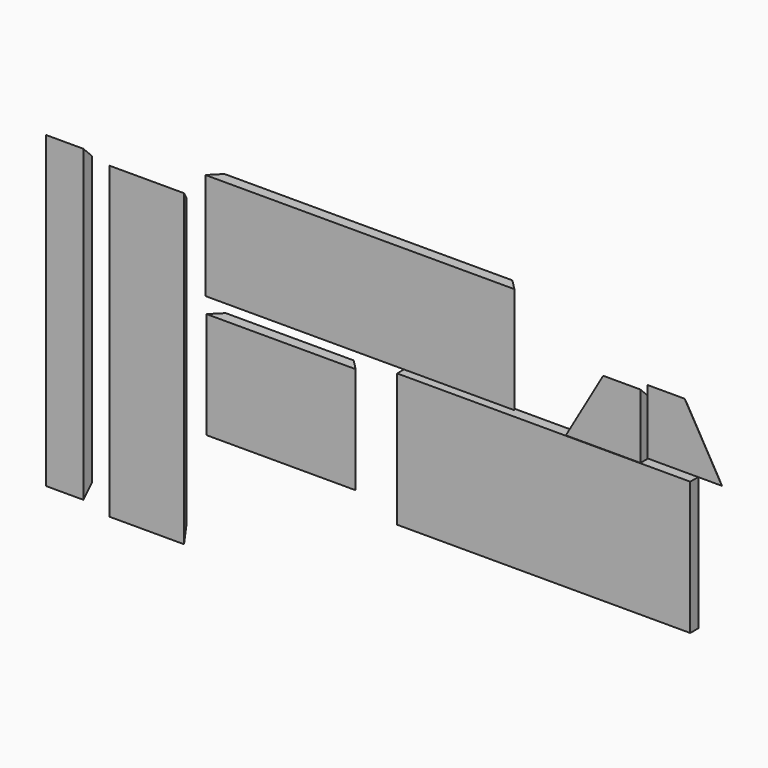
from build123d import *

# Parameters (mm, degrees)
F0_W      = 368.3
F0_H      = 127
F1_DEPTH  = 12.7
F2_W      = 177.8
F2_H      = 127
F3_DEPTH  = 12.7
F4_SIZE   = 12.69999
F5_SIZE   = 12.69999
F6_W      = 3.175
F6_H      = 12.7
F7_DEPTH  = 368.3
F8_W      = 3.175
F8_H      = 12.7
F9_DEPTH  = 368.3
F10_SIZE  = 12.69999
F11_SIZE  = 12.69999
F12_W     = 349.25
F12_H     = 158.75
F13_DEPTH = 12.7
F14_W     = 44.45
F14_H     = 368.3
F15_DEPTH = 12.7
F17_DEPTH = 12.7
F18_SIZE  = 12.69999
F20_DEPTH = 368.3
F21_SIZE  = 12.69999
F22_W     = 88.9
F22_H     = 368.3
F23_DEPTH = 12.7
F25_DEPTH = 368.3
F27_DEPTH = 12.7
F28_SIZE  = 12.69999
F29_SIZE  = 12.69999


# Not quite as in the source:
# - a fillet or chamfer is up to 0.001 mm smaller than in the source, because OpenCascade refuses the exact size
# - a feature names something its author has since deleted; it is built from what else it names


with BuildPart() as f1:
    # F0 (on Front) → F1 (new body)
    with BuildSketch(Plane.XZ):
        with Locations((-48.202611506, 52.6261187441)):
            Rectangle(F0_W, F0_H)
    extrude(amount=F1_DEPTH)

    # F4 (size 12.7 in the source; OpenCascade refuses exactly that, so slightly less here)
    f4_edges = [f1.edges().sort_by_distance(p)[0] for p in [
        (135.947388, 0, 52.626119),
    ]]
    chamfer(f4_edges, length=F4_SIZE)

    # F6 (on face) → F7 (cut)
    with BuildSketch(Plane(origin=(-232.352611506, 0, 0), x_dir=(0, -1, 0), z_dir=(-1, 0, 0))):
        with Locations((1.5875, -4.5238812559)):
            Rectangle(F6_W, F6_H)
    extrude(amount=-F7_DEPTH, mode=Mode.SUBTRACT)

    # F10 (size 12.7 in the source; OpenCascade refuses exactly that, so slightly less here)
    f10_edges = [f1.edges().sort_by_distance(p)[0] for p in [
        (-232.352612, 0, 58.976119),
    ]]
    chamfer(f10_edges, length=F10_SIZE)


with BuildPart() as f3:
    # F2 (on Front) → F3 (new body)
    with BuildSketch(Plane.XZ):
        with Locations((-142.0882418752, -92.8593969557)):
            Rectangle(F2_W, F2_H)
    extrude(amount=F3_DEPTH)

    # F5 (size 12.7 in the source; OpenCascade refuses exactly that, so slightly less here)
    f5_edges = [f3.edges().sort_by_distance(p)[0] for p in [
        (-53.188242, 0, -92.859397),
    ]]
    chamfer(f5_edges, length=F5_SIZE)

    # F8 (on face) → F9 (cut)
    with BuildSketch(Plane(origin=(-230.9882418752, 0, 0), x_dir=(0, -1, 0), z_dir=(-1, 0, 0))):
        with Locations((1.5875, -150.0093969557)):
            Rectangle(F8_W, F8_H)
    extrude(amount=-F9_DEPTH, mode=Mode.SUBTRACT)

    # F11 (size 12.7 in the source; OpenCascade refuses exactly that, so slightly less here)
    f11_edges = [f3.edges().sort_by_distance(p)[0] for p in [
        (-230.988242, 0, -86.509397),
    ]]
    chamfer(f11_edges, length=F11_SIZE)


with BuildPart() as f13:
    # F12 (on Front) → F13 (new body)
    with BuildSketch(Plane.XZ):
        with Locations((170.78008526, -97.0997214928)):
            Rectangle(F12_W, F12_H)
    extrude(amount=F13_DEPTH)


with BuildPart() as f15:
    # F14 (on Front) → F15 (new body)
    with BuildSketch(Plane.XZ):
        with Locations((-399.9289679691, -87.7866384085)):
            Rectangle(F14_W, F14_H)
    extrude(amount=F15_DEPTH)

    # F19 (on face) → F20 (cut)
    with BuildSketch(Plane(origin=(0, 0, -271.9366384085), x_dir=(1, 0, 0), z_dir=(0, 0, -1))):
        Polygon((-414.8216195504, 0), (-422.1539679691, 12.7), (-422.1539679691, 0), align=None)
    extrude(amount=-F20_DEPTH, mode=Mode.SUBTRACT)

    # F21 (size 12.7 in the source; OpenCascade refuses exactly that, so slightly less here)
    f21_edges = [f15.edges().sort_by_distance(p)[0] for p in [
        (-396.262794, 0, 96.363362),
        (-396.262794, 0, -271.936638),
    ]]
    chamfer(f21_edges, length=F21_SIZE)


with BuildPart() as f17:
    # F16 (on Front) → F17 (new body)
    with BuildSketch(Plane.XZ):
        Polygon((294.2917943001, 67.1830539138), (294.2917943001, -9.8066044826), (383.1917943001, -9.8066044826), (338.7417943001, 67.1830539138), align=None)
    extrude(amount=F17_DEPTH)

    # F18 (size 12.7 in the source; OpenCascade refuses exactly that, so slightly less here)
    f18_edges = [f17.edges().sort_by_distance(p)[0] for p in [
        (360.966794, 0, 28.688225),
        (316.516794, 0, 67.183054),
    ]]
    chamfer(f18_edges, length=F18_SIZE)


with BuildPart() as f23:
    # F22 (on Front) → F23 (new body)
    with BuildSketch(Plane.XZ):
        with Locations((-302.1833447643, -95.3806303442)):
            Rectangle(F22_W, F22_H)
    extrude(amount=F23_DEPTH)

    # F24 (on face) → F25 (cut)
    with BuildSketch(Plane.XY.offset(88.7693696558)):
        Polygon((-346.6333447643, 0), (-346.6333447643, -12.7), (-339.3009963456, 0), align=None)
        Polygon((-265.065693183, 0), (-257.7333447643, -12.7), (-257.7333447643, 0), align=None)
    extrude(amount=-F25_DEPTH, mode=Mode.SUBTRACT)

    # F29 (size 12.7 in the source; OpenCascade refuses exactly that, so slightly less here)
    f29_edges = [f23.edges().sort_by_distance(p)[0] for p in [
        (-302.183345, 0, 88.76937),
        (-302.183345, 0, -279.53063),
    ]]
    chamfer(f29_edges, length=F29_SIZE)


with BuildPart() as f27:
    # F26 (on Front) → F27 (new body)
    with BuildSketch(Plane.XZ):
        Polygon((197.2266658425, -17.2972651758), (286.1266658425, -17.2972651758), (286.1266658425, 59.6923932206), (241.6766658425, 59.6923932206), align=None)
    extrude(amount=F27_DEPTH)

    # F28 (size 12.7 in the source; OpenCascade refuses exactly that, so slightly less here)
    f28_edges = [f27.edges().sort_by_distance(p)[0] for p in [
        (219.451666, 0, 21.197564),
        (263.901666, 0, 59.692393),
    ]]
    chamfer(f28_edges, length=F28_SIZE)


solid = Compound([f1.part, f3.part, f13.part, f15.part, f17.part, f23.part, f27.part])
